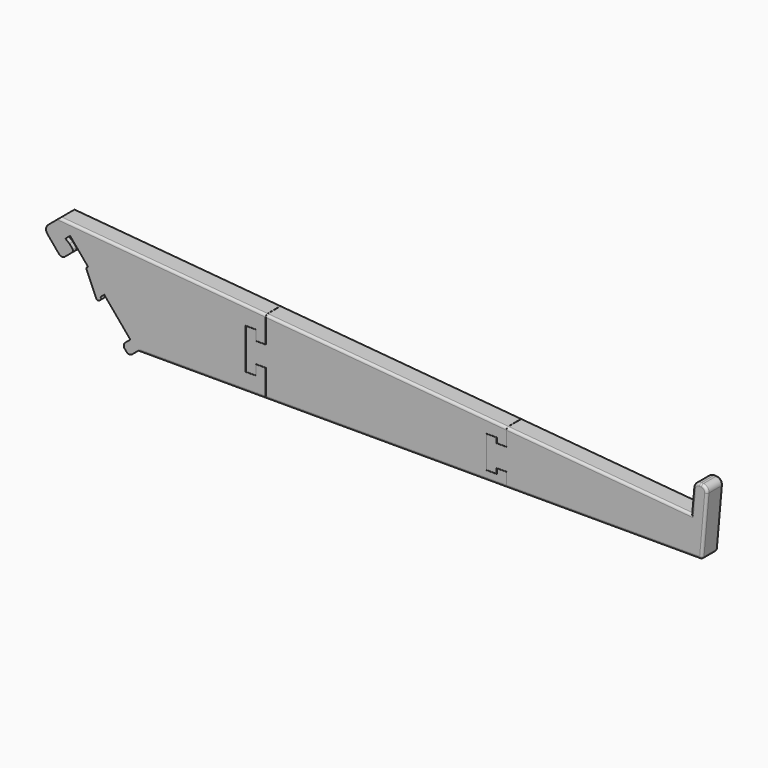
from build123d import *

# Parameters (mm, degrees)
F1_DEPTH         = 12.7
F2_W             = 13.335
F2_H             = 7.0866
F3_DEPTH         = 93.472
F5_DEPTH         = 25.4
F7_R             = 1.524
F10_F1_R         = 1.524
F10_F2_R         = 1.524
F10_S1_F1_R      = 1.524
F10_S1_F2_R      = 1.524
F10_S2_T1_DEPTH  = 126.041432676
F10_S2_T3_DEPTH  = 1.27
F10_S2_T5_DEPTH  = 36.5738786888
F10_S2_T7_DEPTH  = 121.0088094258
F10_S2_T9_DEPTH  = 15.24
F10_S2_T11_DEPTH = 9.652
F10_S2_T16_DEPTH = 1.524
F10_S2_T22_DEPTH = 1.524
F10_S2_T26_ANGLE = 90
F10_S2_T28_ANGLE = 90
F10_S2_T33_DEPTH = 124.8188094258
F10_S2_T37_DEPTH = 19.05


# Not quite as in the source:
# - a fillet or chamfer that OpenCascade refuses, or shapes differently, is made with other operations: its cross-section is extruded or revolved along the edge and cut away or added
# - a feature of the source that left no trace in its solid (it failed there, or was rolled back) is left out


with BuildPart() as f1:
    # F0 (on Front) → F1 (new body)
    with BuildSketch(Plane.XZ):
        with BuildLine():
            ThreePointArc((-46.0617865298, -15.3783926414), (-47.4082675367, -17.9649585898), (-46.5313950652, -20.7460427626))
            Line((-46.5313950652, -20.7460427626), (-39.1843326865, -29.5019307475))
            ThreePointArc((-39.1843326865, -29.5019307475), (-37.4599553875, -30.399584752), (-35.6058992724, -29.8150031044))
            Line((-35.6058992724, -29.8150031044), (-30.7415170586, -25.7333017829))
            ThreePointArc((-30.7415170586, -25.7333017829), (-30.2926900563, -24.8711131334), (-30.5849808801, -23.9440850758))
            Line((-30.5849808801, -23.9440850758), (-32.6258315409, -21.5118939689))
            Line((-32.6258315409, -21.5118939689), (-35.2214163384, -19.5451800716))
            Line((-35.2214163384, -19.5451800716), (-32.2344910947, -17.0388522013))
            Line((-32.2344910947, -17.0388522013), (-20.8873614209, -30.5618347556))
            Line((-20.8873614209, -30.5618347556), (-21.3737996423, -30.9700048878))
            ThreePointArc((-21.3737996423, -30.9700048878), (-21.7934146066, -31.6507945747), (-21.722945379, -32.4474032641))
            Line((-21.722945379, -32.4474032641), (-15.4658563045, -46.9017792559))
            ThreePointArc((-15.4658563045, -46.9017792559), (-14.603667655, -47.3506062582), (-13.6766395974, -47.0583154344))
            Line((-13.6766395974, -47.0583154344), (-12.2173249333, -45.8338050379))
            Line((-12.2173249333, -45.8338050379), (-13.0336651976, -44.8609285952))
            Line((-13.0336651976, -44.8609285952), (-10.6014740907, -42.8200779344))
            Line((-10.6014740907, -42.8200779344), (5.8885992482, -62.4721820782))
            Line((5.8885992482, -62.4721820782), (2.6781069871, -65.1661049504))
            ThreePointArc((2.6781069871, -65.1661049504), (1.7804529825, -66.8904822493), (2.3650346302, -68.7445383645))
            Line((2.3650346302, -68.7445383645), (3.4262769738, -70.0092777401))
            ThreePointArc((3.4262769738, -70.0092777401), (5.1506542727, -70.9069317447), (7.0047103879, -70.322350097))
            Line((7.0047103879, -70.322350097), (10.215202649, -67.6284272248))
            Line((10.215202649, -67.6284272248), (367.6347867909, -67.6284272248))
            Line((367.6347867909, -67.6284272248), (370.9441223638, -29.8025485384))
            ThreePointArc((370.9441223638, -29.8025485384), (370.0672498924, -27.0214643656), (367.480683944, -25.6749833588))
            Line((367.480683944, -25.6749833588), (366.2155166774, -25.5642955655))
            ThreePointArc((366.2155166774, -25.5642955655), (363.4344325046, -26.4411680369), (362.0879514978, -29.0277339854))
            Line((362.0879514978, -29.0277339854), (360.7596979783, -44.2097411843))
            Line((360.7596979783, -44.2097411843), (-38.7652132091, -9.2558406592))
            Line((-38.7652132091, -9.2558406592), (-46.0617865298, -15.3783926414))
        make_face()
    extrude(amount=F1_DEPTH)

    # F2 (on face) → F3 (cut)
    with BuildSketch(Plane(origin=(-11.4592404683, 0, 13.6565909966), x_dir=(0.7660444431, 0, 0.6427876097), z_dir=(-0.6427876097, 0, 0.7660444431))):
        with Locations((-42.3129158581, -6.3627)):
            Rectangle(F2_W, F2_H)
    extrude(amount=-F3_DEPTH, mode=Mode.SUBTRACT)

    # F4 (on face) → F5 (cut)
    with BuildSketch(Plane.XZ.offset(12.7)):
        Polygon((91.5814654057, -20.6596973662), (91.6830654057, -20.6685862144), (91.6830654057, 1.1655155965), (91.5814654057, 1.1653002073), align=None)
        Polygon((91.5814654057, -67.6284272248), (91.6830654057, -67.6284272248), (91.6830654057, -50.2417070188), (85.3330660997, -50.2417070188), (85.3330660997, -56.5917070188), (78.9830660997, -56.5917070188), (78.9830660997, -31.0393070188), (85.3330660997, -31.0393070188), (85.3330660997, -37.3893070188), (91.6830654057, -37.3893070188), (91.6830654057, -20.6685862144), (91.5814654057, -20.6596973662), (91.5814654057, -37.2877070188), (85.4346660997, -37.2877070188), (85.4346660997, -30.9377070188), (78.8814660997, -30.9377070188), (78.8814660997, -56.6933070188), (85.5108660997, -56.6933070188), (85.5108660997, -50.3433070188), (91.5814654057, -50.3433070188), align=None)
        Polygon((243.9052654057, -33.9863030514), (244.0068654057, -33.9951918996), (244.0068654057, -9.7616507337), (243.9052654057, -9.7616507337), align=None)
        Polygon((243.9052654057, -58.7221217398), (243.9052654057, -67.6284272248), (244.0068654057, -67.6284272248), (244.0068654057, -58.6205217398), (237.7330654057, -58.6205217398), (237.7330654057, -61.8209217398), (231.3830654057, -61.8209217398), (231.3830654057, -41.6279271885), (237.7330654057, -41.6279271885), (237.7330654057, -44.8283271885), (244.0068654057, -44.8283271885), (244.0068654057, -33.9951918996), (243.9052654057, -33.9863030514), (243.9052654057, -44.7267271885), (237.8346654057, -44.7267271885), (237.8346654057, -41.5263271885), (231.2814654057, -41.5263271885), (231.2814654057, -61.9225217398), (237.8346654057, -61.9225217398), (237.8346654057, -58.7221217398), align=None)
    extrude(amount=-F5_DEPTH, mode=Mode.SUBTRACT)

    # F7
    f7_edges = [f1.edges().sort_by_distance(p)[0] for p in [
        (26.408126, -12.7, -14.957769),
        (167.794165, -12.7, -27.327445),
        (302.383282, -12.7, -39.102467),
        (361.423825, -12.7, -36.618738),
        (167.794165, -12.7, -67.628427),
        (50.898334, -12.7, -67.628427),
    ]]
    fillet(f7_edges, radius=F7_R)

    # F10: fillet of radius 1.524 on 2 edges, made by hand

    # F10_f1
    f10_f1_edges = [f1.edges().sort_by_distance(p)[0] for p in [
        (26.4081260983, 0, -14.9577690127),
    ]]
    fillet(f10_f1_edges, radius=F10_F1_R)

    # F10_f2
    f10_f2_edges = [f1.edges().sort_by_distance(p)[0] for p in [
        (50.8983340273, 0, -67.6284272248),
    ]]
    fillet(f10_f2_edges, radius=F10_F2_R)

    # F10#s1: fillet of radius 1.524 on 2 edges, made by hand

    # F10_s1_f1
    f10_s1_f1_edges = [f1.edges().sort_by_distance(p)[0] for p in [
        (167.7941654057, 0, -27.3274446329),
    ]]
    fillet(f10_s1_f1_edges, radius=F10_S1_F1_R)

    # F10_s1_f2
    f10_s1_f2_edges = [f1.edges().sort_by_distance(p)[0] for p in [
        (167.7941654057, 0, -67.6284272248),
    ]]
    fillet(f10_s1_f2_edges, radius=F10_S1_F2_R)

    # F10#s2: fillet of radius 1.524 on 9 edges, made by hand

    # F10_s2_s2 → F10_s2_t1 (cut)
    with BuildSketch(Plane.YZ.offset(240.1968654057)):
        with BuildLine():
            ThreePointArc((-12.7, -66.1044272248), (-12.2536307345, -67.1820579594), (-11.176, -67.6284272248))
            Line((-11.176, -67.6284272248), (-12.7, -67.6284272248))
            Line((-12.7, -67.6284272248), (-12.7, -66.1044272248))
        make_face()
        with BuildLine():
            ThreePointArc((0, -66.1044272248), (-0.4463692655, -67.1820579594), (-1.524, -67.6284272248))
            Line((-1.524, -67.6284272248), (0, -67.6284272248))
            Line((0, -67.6284272248), (0, -66.1044272248))
        make_face()
    extrude(amount=F10_S2_T1_DEPTH, mode=Mode.SUBTRACT)

    # F10_s2_s4 → F10_s2_t3 (cut)
    with BuildSketch(Plane(origin=(366.9184623231, 0, -32.1012058916), x_dir=(0, 1, 0), z_dir=(-0.9961946981, 0, 0.0871557427))):
        with BuildLine():
            ThreePointArc((-1.524, -6.4507696589), (-0.4463692655, -6.0044003935), (0, -4.9267696589))
            Line((0, -4.9267696589), (0, -6.4507696589))
            Line((0, -6.4507696589), (-1.524, -6.4507696589))
        make_face()
    extrude(amount=F10_S2_T3_DEPTH, mode=Mode.SUBTRACT)

    # F10_s2_s6 → F10_s2_t5 (cut)
    with BuildSketch(Plane(origin=(-2.9574653212, 0, -33.8039833053), x_dir=(0, 1, 0), z_dir=(0.0871557427, 0, 0.9961946981))):
        with BuildLine():
            ThreePointArc((0, -370.6060312408), (-0.4463692655, -371.6836619753), (-1.524, -372.1300312408))
            Line((-1.524, -372.1300312408), (0, -372.1300312408))
            Line((0, -372.1300312408), (0, -370.6060312408))
        make_face()
    extrude(amount=F10_S2_T5_DEPTH, mode=Mode.SUBTRACT)

    # F10_s2_s8 → F10_s2_t7 (cut)
    with BuildSketch(Plane(origin=(361.8577932568, 0, -31.6584547185), x_dir=(0, 1, 0), z_dir=(-0.9961946981, 0, 0.0871557427))):
        with BuildLine():
            ThreePointArc((0, 14.1232303411), (-0.4463692655, 13.0455996065), (-1.524, 12.5992303411))
            Line((-1.524, 12.5992303411), (0, 12.5992303411))
            Line((0, 12.5992303411), (0, 14.1232303411))
        make_face()
    extrude(amount=F10_S2_T7_DEPTH, mode=Mode.SUBTRACT)

    # F10_s2_s10 → F10_s2_t9 (cut)
    with BuildSketch(Plane(origin=(0.2301582411, 0, 2.6307207331), x_dir=(0, 1, 0), z_dir=(-0.0871557427, 0, -0.9961946981))):
        with BuildLine():
            ThreePointArc((0, 364.7640312408), (-0.4463692655, 363.6864005063), (-1.524, 363.2400312408))
            Line((-1.524, 363.2400312408), (0, 363.2400312408))
            Line((0, 363.2400312408), (0, 364.7640312408))
        make_face()
    extrude(amount=F10_S2_T9_DEPTH, mode=Mode.SUBTRACT)

    # F10_s2_s12 → F10_s2_t11 (cut)
    with BuildSketch(Plane.XZ.offset(1.524)):
        with BuildLine():
            ThreePointArc((367.7564988016, -66.2372525768), (367.2678975581, -67.2280378861), (366.2382980817, -67.6284272248))
            Line((366.2382980817, -67.6284272248), (367.6347867909, -67.6284272248))
            Line((367.6347867909, -67.6284272248), (367.7564988016, -66.2372525768))
        make_face()
    extrude(amount=F10_S2_T11_DEPTH, mode=Mode.SUBTRACT)


with BuildPart() as f10_s2_tool14:
    # F10_s2_s15 → F10_s2_t16 (new body)
    with BuildSketch(Plane.XZ.offset(11.176)):
        Polygon((366.2382980817, -66.1044272248), (367.7564988016, -66.2372525768), (367.6347867909, -67.6284272248), (366.2382980817, -67.6284272248), align=None)
    extrude(amount=F10_S2_T16_DEPTH)

    # F10_s2_s17 → F10_s2_t18 (revolve, cut)
    with BuildSketch(Plane(origin=(366.2382980817, -11.176, -66.1044272248), x_dir=(-0.6755902076, 0, 0.7372773368), z_dir=(0.7372773368, 0, 0.6755902076))):
        with BuildLine():
            ThreePointArc((0, -1.524), (1.524, 0), (0, 1.524))
            Line((0, 1.524), (0, -1.524))
        make_face()
    revolve(axis=Axis((366.2382980817, -11.176, -66.1044272248), (0, -1, 0)), mode=Mode.SUBTRACT)


with BuildPart() as f1_1:
    add(f1.part)

    # F10_s2_t13: cut F10_s2_tool14
    add(f10_s2_tool14.part, mode=Mode.SUBTRACT)


with BuildPart() as f10_s2_tool20:
    # F10_s2_s21 → F10_s2_t22 (new body)
    with BuildSketch(Plane.XZ.offset(1.524)):
        Polygon((366.2382980817, -66.1044272248), (367.7564988016, -66.2372525768), (367.6347867909, -67.6284272248), (366.2382980817, -67.6284272248), align=None)
    extrude(amount=-F10_S2_T22_DEPTH)

    # F10_s2_s23 → F10_s2_t24 (revolve, cut)
    with BuildSketch(Plane(origin=(366.2382980817, -1.524, -66.1044272248), x_dir=(-0.6755902076, 0, 0.7372773368), z_dir=(-0.7372773368, 0, -0.6755902076))):
        with BuildLine():
            ThreePointArc((0, -1.524), (1.524, 0), (0, 1.524))
            Line((0, 1.524), (0, -1.524))
        make_face()
    revolve(axis=Axis((366.2382980817, -1.524, -66.1044272248), (0, 1, 0)), mode=Mode.SUBTRACT)


with BuildPart() as f1_2:
    add(f1_1.part)

    # F10_s2_t19: cut F10_s2_tool20
    add(f10_s2_tool20.part, mode=Mode.SUBTRACT)

    # F10_s2_s25 → F10_s2_t26 (revolve, cut)
    with BuildSketch(Plane(origin=(365.6532950565, 0, -31.9905180983), x_dir=(0, 1, 0), z_dir=(0.9961946981, 0, -0.0871557427))):
        with BuildLine():
            ThreePointArc((-1.524, 6.4507696589), (-0.4463692655, 6.0044003935), (0, 4.9267696589))
            Line((0, 4.9267696589), (0, 6.4507696589))
            Line((0, 6.4507696589), (-1.524, 6.4507696589))
        make_face()
    revolve(axis=Axis((365.8834532975, 0, -29.3597973652), (0, -1, 0)), revolution_arc=F10_S2_T26_ANGLE, mode=Mode.SUBTRACT)

    # F10_s2_s27 → F10_s2_t28 (revolve, cut)
    with BuildSketch(Plane(origin=(0.2301582411, 0, 2.6307207331), x_dir=(0, 1, 0), z_dir=(-0.0871557427, 0, -0.9961946981))):
        with BuildLine():
            ThreePointArc((0, 370.6060312408), (-0.4463692655, 371.6836619753), (-1.524, 372.1300312408))
            Line((-1.524, 372.1300312408), (0, 372.1300312408))
            Line((0, 372.1300312408), (0, 370.6060312408))
        make_face()
    revolve(axis=Axis((367.1486205641, 0, -29.4704851585), (0, -1, 0)), revolution_arc=F10_S2_T28_ANGLE, mode=Mode.SUBTRACT)


with BuildPart() as f10_s2_tool31:
    # F10_s2_s32 → F10_s2_t33 (new body)
    with BuildSketch(Plane(origin=(365.6532950565, 0, -31.9905180983), x_dir=(0, 1, 0), z_dir=(-0.9961946981, 0, 0.0871557427))):
        with BuildLine():
            ThreePointArc((0, 14.1232303411), (-0.4463692655, 13.0455996065), (-1.524, 12.5992303411))
            Line((-1.524, 12.5992303411), (0, 12.5992303411))
            Line((0, 12.5992303411), (0, 14.1232303411))
        make_face()
    extrude(amount=F10_S2_T33_DEPTH)

    split(bisect_by=Plane(origin=(361.8577932568, 0, -31.6584547185), x_dir=(0, 1, 0), z_dir=(0.9961946981, 0, -0.0871557427)), keep=Keep.TOP)


with BuildPart() as f10_s2_tool35:
    # F10_s2_s36 → F10_s2_t37 (new body)
    with BuildSketch(Plane(origin=(0.2301582411, 0, 2.6307207331), x_dir=(0, 1, 0), z_dir=(-0.0871557427, 0, -0.9961946981))):
        with BuildLine():
            ThreePointArc((0, 364.7640312408), (-0.4463692655, 363.6864005063), (-1.524, 363.2400312408))
            Line((-1.524, 363.2400312408), (0, 363.2400312408))
            Line((0, 363.2400312408), (0, 364.7640312408))
        make_face()
    extrude(amount=F10_S2_T37_DEPTH)

    split(bisect_by=Plane(origin=(-1.0980952784, 0, -12.5512864658), x_dir=(0, 1, 0), z_dir=(-0.0871557427, 0, -0.9961946981)), keep=Keep.TOP)


with BuildPart() as f10_s2_tool31_1:
    add(f10_s2_tool31.part)

    # F10_s2_t39: intersect F10_s2_tool35
    add(f10_s2_tool35.part, mode=Mode.INTERSECT)


with BuildPart() as f1_3:
    add(f1_2.part)

    # F10_s2_t29: cut F10_s2_tool31
    add(f10_s2_tool31_1.part, mode=Mode.SUBTRACT)


solid = f1_3.part
